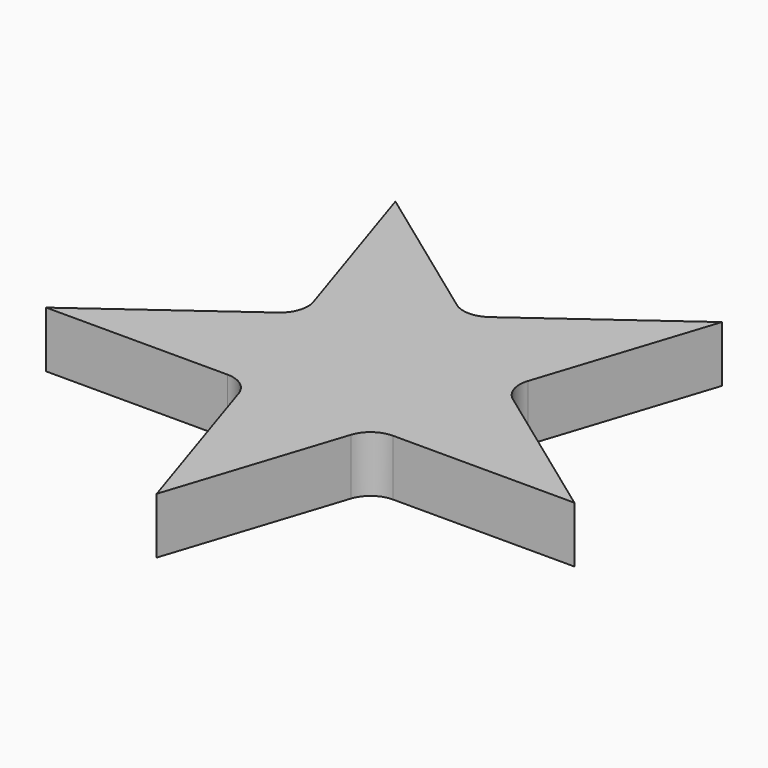
from build123d import *

# Parameters (mm, degrees)
F1_DEPTH = 10
F3_START = -1.5
F3_DEPTH = 7
F4_R     = 5


with BuildPart() as f1:
    # F0 (on Top) → F1 (new body)
    with BuildSketch(Plane.XY):
        Polygon((0, 18.8854382), (-29.0617011202, 40), (-17.9611190632, 5.83592135), align=None)
        Polygon((17.9611190632, 5.83592135), (29.0617011202, 40), (0, 18.8854382), align=None)
        Polygon((0, 18.8854382), (-17.9611190632, 5.83592135), (-11.100582057, -15.27864045), (11.100582057, -15.27864045), (17.9611190632, 5.83592135), align=None)
        Polygon((11.100582057, -15.27864045), (47.0228201834, -15.27864045), (17.9611190632, 5.83592135), align=None)
        Polygon((-11.100582057, -15.27864045), (0, -49.4427191), (11.100582057, -15.27864045), align=None)
        Polygon((-17.9611190632, 5.83592135), (-47.0228201834, -15.27864045), (-11.100582057, -15.27864045), align=None)
    extrude(amount=F1_DEPTH)

    # F2 (on face) → F3 (cut)
    with BuildSketch(Plane.XY.offset(10).offset(F3_START)):
        Polygon((-9.25, -11.1145618), (0, -11.1145618), (9.25, -11.1145618), (9.25, 25.605956584), (0, 18.8854382), (-9.25, 25.605956584), align=None)
    extrude(amount=-F3_DEPTH, mode=Mode.SUBTRACT)

    # F4
    f4_edges = [f1.edges().sort_by_distance(p)[0] for p in [
        (-17.961119, 5.835921, 5),
        (-11.100582, -15.27864, 5),
        (11.100582, -15.27864, 5),
        (17.961119, 5.835921, 5),
        (0, 18.885438, 9.25),
        (0, 18.885438, 0.75),
        (9.25, 25.605957, 5),
        (-9.25, 25.605957, 5),
    ]]
    fillet(f4_edges, radius=F4_R)


solid = f1.part
